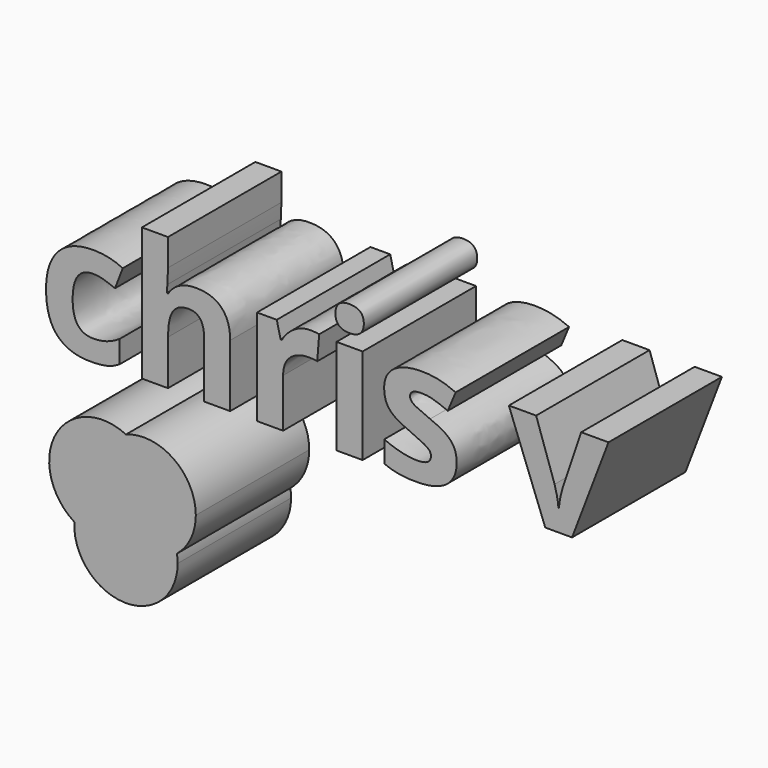
from build123d import *

# Parameters (mm, degrees)
F0_TEXT_SIZE = 31.3733684986
F1_DEPTH     = 25.4
F3_DEPTH     = 25.4


# Not quite as in the source:
# - Text() gives the source's letters only with a copy of the font that has no kerning and outlines rounded to 1/6400 em; it was checked with that copy


with BuildPart() as f1:
    # F0 (on Front) → F1 (new body)
    with BuildSketch(Plane.XZ):
        with Locations((-46.886049211, -6.3590393402)):
            Text('chris v', F0_TEXT_SIZE, font='Open Sans', font_style=FontStyle.BOLD, text_align=(TextAlign.LEFT, TextAlign.BOTTOM))
    extrude(amount=F1_DEPTH)


with BuildPart() as f3:
    # F2 (on Front) → F3 (new body)
    with BuildSketch(Plane.XZ):
        with BuildLine():
            ThreePointArc((-37.036101516, -26.2840416865), (-35.9202354295, -20.1433315897), (-31.1600198782, -16.1067704887))
            ThreePointArc((-31.1600198782, -16.1067704887), (-43.7245350763, -20.1433315897), (-40.402215221, -32.9152953566))
            ThreePointArc((-40.402215221, -32.9152953566), (-39.4143494103, -29.2467801825), (-37.036101516, -26.2840416865))
        make_face()
        with BuildLine():
            ThreePointArc((-25.7686132946, -25.9119724209), (-25.7176982897, -25.342886287), (-25.7007065845, -24.7717797756))
            ThreePointArc((-25.7007065845, -24.7717797756), (-27.1793331289, -19.651074561), (-31.1600198782, -16.1067704887))
            ThreePointArc((-31.1600198782, -16.1067704887), (-35.9202354295, -20.1433315897), (-37.036101516, -26.2840416865))
            ThreePointArc((-37.036101516, -26.2840416865), (-31.4655298808, -24.1849355143), (-25.7686132946, -25.9119724209))
        make_face()
        with BuildLine():
            ThreePointArc((-31.1600198782, -16.1067704887), (-27.1793331289, -19.651074561), (-25.7007065845, -24.7717797756))
            ThreePointArc((-25.7007065845, -24.7717797756), (-25.7176982897, -25.342886287), (-25.7686132946, -25.9119724209))
            ThreePointArc((-25.7686132946, -25.9119724209), (-23.3005180613, -28.546148856), (-22.0275697065, -31.9240153511))
            ThreePointArc((-22.0275697065, -31.9240153511), (-19.5348675631, -28.7271948409), (-18.6472206673, -24.7717797756))
            ThreePointArc((-18.6472206673, -24.7717797756), (-22.6339350452, -17.161711937), (-31.1600198782, -16.1067704887))
        make_face()
        with BuildLine():
            ThreePointArc((-31.1600198782, -33.4367890625), (-27.4981449445, -30.3666267324), (-25.7686132946, -25.9119724209))
            ThreePointArc((-25.7686132946, -25.9119724209), (-31.4655298808, -24.1849355143), (-37.036101516, -26.2840416865))
            ThreePointArc((-37.036101516, -26.2840416865), (-35.0563798172, -30.6476878852), (-31.1600198782, -33.4367890625))
        make_face()
        with BuildLine():
            ThreePointArc((-37.036101516, -26.2840416865), (-39.4143494103, -29.2467801825), (-40.402215221, -32.9152953566))
            ThreePointArc((-40.402215221, -32.9152953566), (-35.8480763147, -34.3627218955), (-31.1600198782, -33.4367890625))
            ThreePointArc((-31.1600198782, -33.4367890625), (-35.0563798172, -30.6476878852), (-37.036101516, -26.2840416865))
        make_face()
        with BuildLine():
            ThreePointArc((-22.0275697065, -31.9240153511), (-23.3005180613, -28.546148856), (-25.7686132946, -25.9119724209))
            ThreePointArc((-25.7686132946, -25.9119724209), (-27.4981449445, -30.3666267324), (-31.1600198782, -33.4367890625))
            ThreePointArc((-31.1600198782, -33.4367890625), (-26.3911146338, -33.9039602542), (-22.0275697065, -31.9240153511))
        make_face()
        with BuildLine():
            ThreePointArc((-31.1600198782, -33.4367890625), (-35.8480763147, -34.3627218955), (-40.402215221, -32.9152953566))
            ThreePointArc((-40.402215221, -32.9152953566), (-31.4208703169, -42.6900094473), (-21.9031235063, -33.4367890625))
            ThreePointArc((-21.9031235063, -33.4367890625), (-21.9342875143, -32.6778471743), (-22.0275697065, -31.9240153511))
            ThreePointArc((-22.0275697065, -31.9240153511), (-26.3911146338, -33.9039602542), (-31.1600198782, -33.4367890625))
        make_face()
    extrude(amount=F3_DEPTH)


solid = Compound([f1.part, f3.part])
